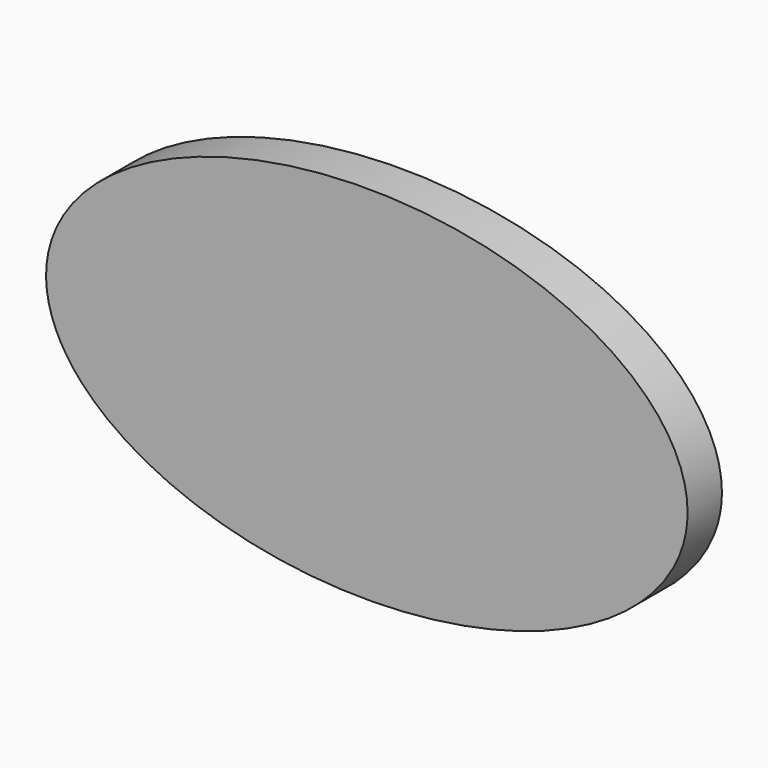
from build123d import *

# Parameters (mm, degrees)
F1_DEPTH = 3.175


# Not quite as in the source:
# - a feature names something its author has since deleted; it is built from what else it names


with BuildPart() as f1:
    # F0 (on Front) → F1 (new body)
    with BuildSketch(Plane.XZ):
        with BuildLine():
            add(Edge.make_bspline(
                [(23.7188442589, 57.1490477352), (23.7188442589, 80.3343560019), (-11.8594221295, 68.7417018686), (-47.4376885178, 57.1490477352), (-11.8594221295, 45.5563936019), (23.7188442589, 33.9637394686), (23.7188442589, 57.1490477352)],
                knots=[0, 0, 0, 2.0943951024, 2.0943951024, 4.1887902048, 4.1887902048, 6.2831853072, 6.2831853072, 6.2831853072], degree=2, weights=[1, 0.5, 1, 0.5, 1, 0.5, 1]))
        make_face()
    extrude(amount=-F1_DEPTH)


solid = f1.part
